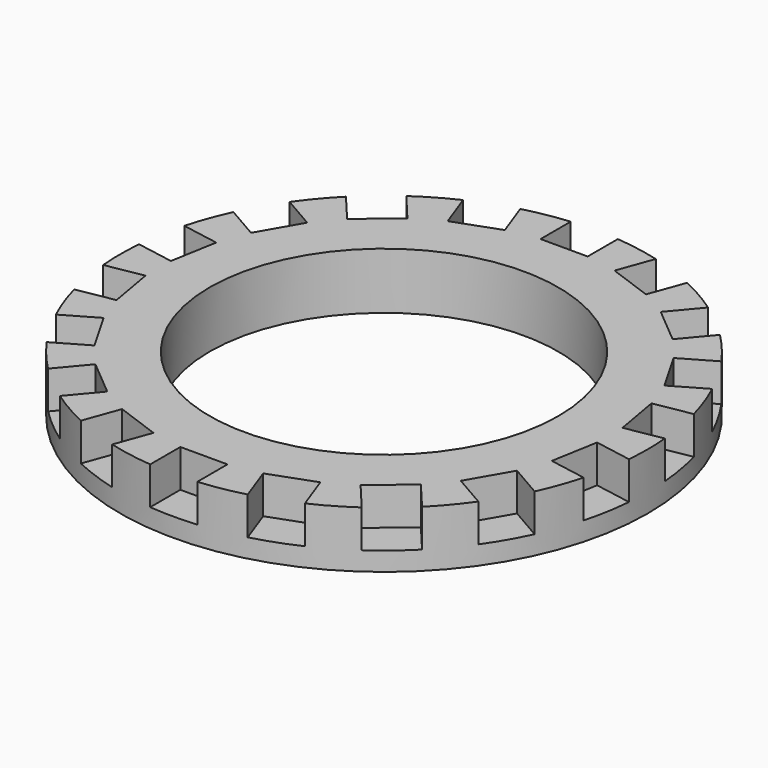
from build123d import *

# Parameters (mm, degrees)
F0_R            = 35.56
F0_R_2          = 23.495
F1_DEPTH        = 7.62
F3_DEPTH        = 5.08
F3_COPIES_COUNT = 18


# Not quite as in the source:
# - a pattern or mirror of a feature is missing from the dataset's text; its kind, count and spacing are read off the source's solid


with BuildPart() as f1:
    # F0 (on Top) → F1 (new body)
    with BuildSketch(Plane.XY):
        Circle(F0_R)
        Circle(F0_R_2, mode=Mode.SUBTRACT)
    extrude(amount=F1_DEPTH)

    # F2 (on face) → F3 (cut)
    with BuildSketch(Plane.XY.offset(7.62)):
        with BuildLine():
            Line((-3.175, -30.3379753092), (-3.175, -35.4179753092))
            ThreePointArc((-3.175, -35.4179753092), (0, -35.56), (3.175, -35.4179753092))
            Line((3.175, -35.4179753092), (3.175, -30.3379753092))
            Line((3.175, -30.3379753092), (-3.175, -30.3379753092))
        make_face()
    f3 = extrude(amount=-F3_DEPTH, mode=Mode.SUBTRACT)

    # F3_copies: F3 ×18 about axis
    f3_copies_axis = Axis((0, 0, 0), (0, 0, 1))
    for i in range(1, F3_COPIES_COUNT):
        add(f3.rotate(f3_copies_axis, i * 360 / F3_COPIES_COUNT), mode=Mode.SUBTRACT)


solid = f1.part
